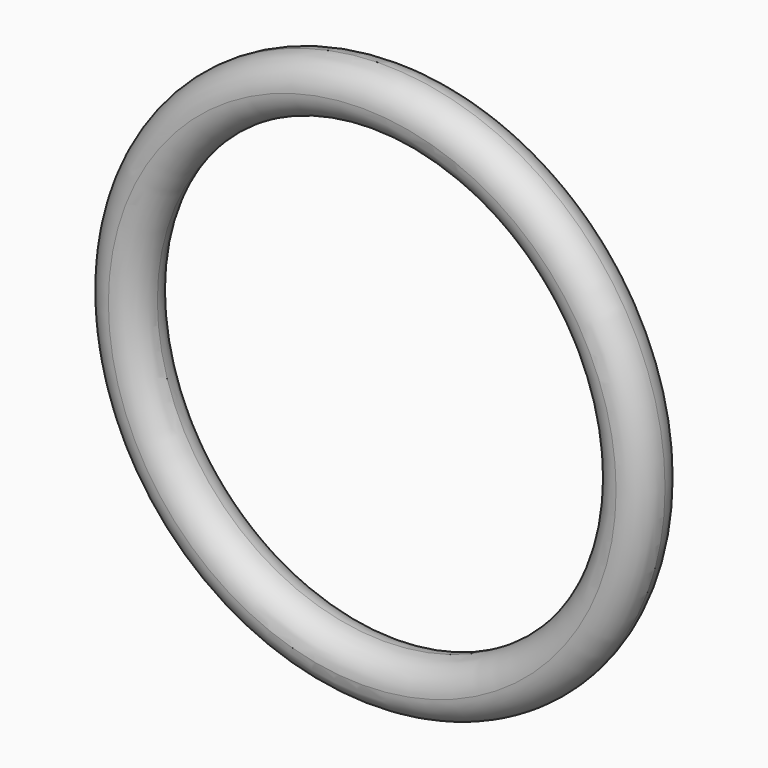
from build123d import *

# Parameters (mm, degrees)
F0_R     = 15.5
F0_R_2   = 12.5
F1_DEPTH = 3
F2_R     = 1.49999


# Not quite as in the source:
# - a fillet or chamfer is up to 0.001 mm smaller than in the source, because OpenCascade refuses the exact size


with BuildPart() as f1:
    # F0 (on Front) → F1 (new body)
    with BuildSketch(Plane.XZ):
        with Locations((-45.8940416574, 28.1622521579)):
            Circle(F0_R)
        with Locations((-45.8940416574, 28.1622521579)):
            Circle(F0_R_2, mode=Mode.SUBTRACT)
    extrude(amount=F1_DEPTH)

    # F2 (radius 1.5 in the source; OpenCascade refuses exactly that, so slightly less here)
    f2_edges = [f1.edges().sort_by_distance(p)[0] for p in [
        (-61.394042, -3, 28.162252),
        (-58.394042, -3, 28.162252),
        (-61.394042, 0, 28.162252),
        (-58.394042, 0, 28.162252),
    ]]
    fillet(f2_edges, radius=F2_R)


solid = f1.part
